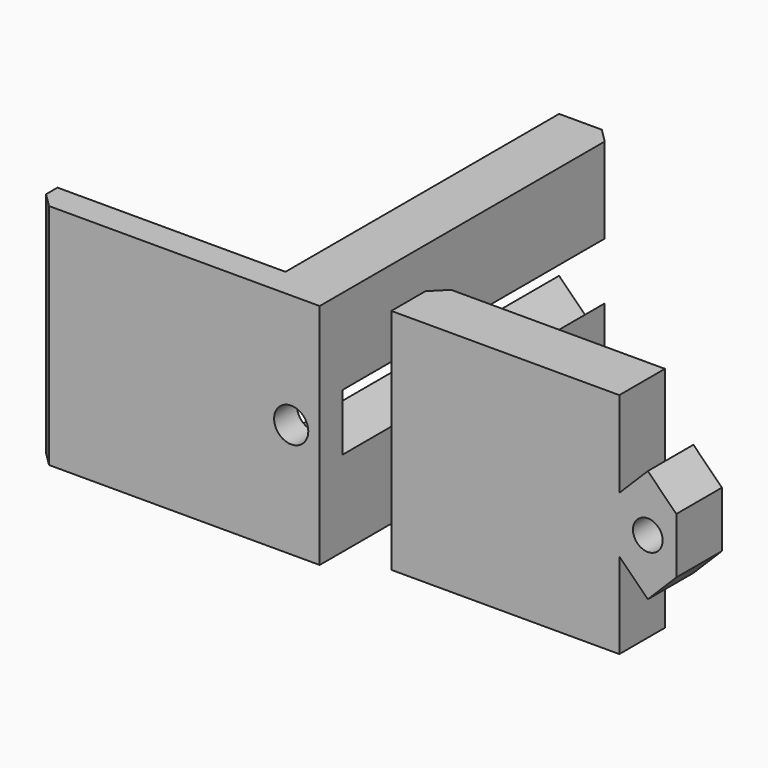
from build123d import *

# Parameters (mm, degrees)
F1_DEPTH  = 50.8
F2_SIZE   = 3.175
F4_DEPTH  = 76.2
F5_R      = 3.81
F6_DEPTH  = 25.8826
F8_DEPTH  = 12.7
F9_R      = 3.302
F10_DEPTH = 14.986
F11_SIZE  = 3.175
F12_ANGLE = 180


with BuildPart() as f1:
    # F0 (on Top) → F1 (new body)
    with BuildSketch(Plane.XY):
        Polygon((0, 76.2), (0, 0), (-50.8, 0), (-50.8, -6.35), (12.7, -6.35), (12.7, 76.2), align=None)
    extrude(amount=F1_DEPTH)

    # F2
    f2_edges = [f1.edges().sort_by_distance(p)[0] for p in [
        (-50.8, -6.35, 25.4),
        (12.7, 76.2, 25.4),
    ]]
    chamfer(f2_edges, length=F2_SIZE)

    # F3 (on Front) → F4 (cut)
    with BuildSketch(Plane.XZ):
        Polygon((0, 31.7502294114), (0, 19.05), (6.35, 12.7), (12.7, 19.05), (12.7, 31.7502294114), (6.4039765843, 38.1), align=None)
    extrude(amount=-F4_DEPTH, mode=Mode.SUBTRACT)

    # F5 (on Front) → F6 (cut)
    with BuildSketch(Plane.XZ):
        with Locations((6.35, 25.4)):
            Circle(F5_R)
    extrude(amount=F6_DEPTH, mode=Mode.SUBTRACT)


with BuildPart() as f8:
    # F7 (on Front) → F8 (new body)
    with BuildSketch(Plane.XZ):
        Polygon((80.7293057442, 37.973), (74.3793057442, 31.623), (74.3793057442, 50.8), (23.5793057442, 50.8), (23.5793057442, 0), (74.3793057442, 0), (74.3793057442, 19.177), (80.7293057442, 12.827), (87.0793057442, 19.177), (87.0793057442, 31.623), align=None)
    extrude(amount=F8_DEPTH)

    # F9 (on Front) → F10 (cut)
    with BuildSketch(Plane.XZ):
        with Locations((80.7293057442, 25.4)):
            Circle(F9_R)
    extrude(amount=F10_DEPTH, mode=Mode.SUBTRACT)

    # F11
    f11_edges = [f8.edges().sort_by_distance(p)[0] for p in [
        (23.579306, -12.7, 25.4),
    ]]
    chamfer(f11_edges, length=F11_SIZE)


with BuildPart() as f8_1:
    # F12: moved
    add(f8.part.rotate(Axis((48.9793057442, 0, 0), (-1, 0, 0)), F12_ANGLE))


with BuildPart() as f8_2:
    # F13: moved
    add(f8_1.part.moved(Location((0, 0, 50.8))))


solid = Compound([f1.part, f8_2.part])
